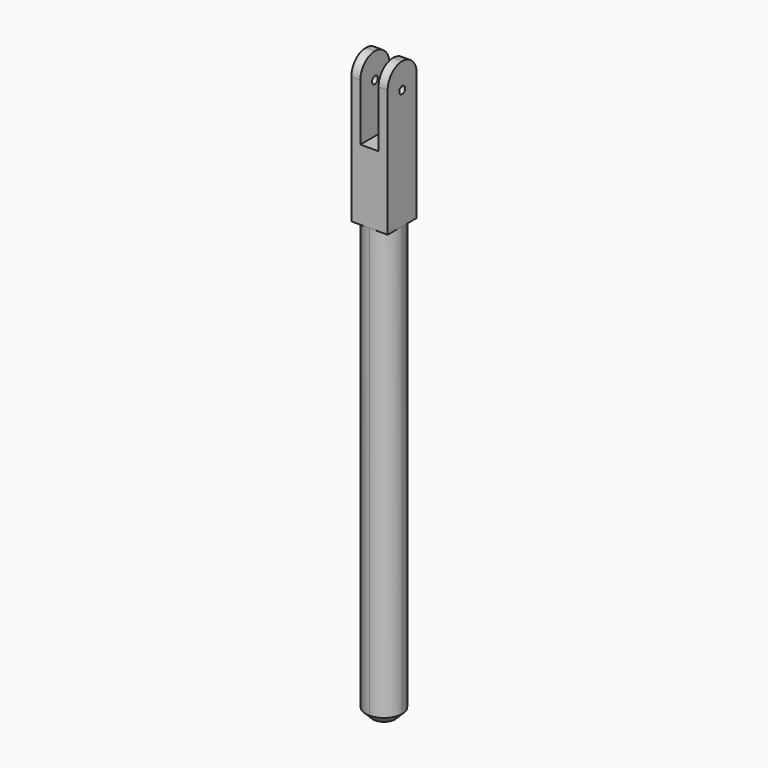
from build123d import *

# Parameters (mm, degrees)
F0_W     = 6.35
F0_H     = 76.2
F1_DEPTH = 3.175
F2_R     = 3.17499
F3_W     = 6.35
F3_H     = 25.4
F5_DEPTH = 3.175
F4_W     = 3.175
F4_H     = 13.0743015936
F6_DEPTH = 5.08
F7_R     = 0.635
F8_DEPTH = 3.81
F9_R     = 3.17499
F10_SIZE = 1.27


# Not quite as in the source:
# - a fillet or chamfer is up to 0.001 mm smaller than in the source, because OpenCascade refuses the exact size


with BuildPart() as f1:
    # F0 (on Front) → F1 (new body, symmetric)
    with BuildSketch(Plane.XZ):
        with Locations((-0.5868453211, -38.1)):
            Rectangle(F0_W, F0_H)
    extrude(amount=F1_DEPTH, both=True)

    # F2 (radius 3.175 in the source; OpenCascade refuses exactly that, so slightly less here)
    f2_edges = [f1.edges().sort_by_distance(p)[0] for p in [
        (2.588155, -3.175, -38.1),
        (2.588155, 3.175, -38.1),
        (-3.761845, -3.175, -38.1),
        (-3.761845, 3.175, -38.1),
    ]]
    fillet(f2_edges, radius=F2_R)

    # F3 (on Front) → F5 (join, symmetric)
    with BuildSketch(Plane.XZ):
        with Locations((-0.5868453211, 12.7)):
            Rectangle(F3_W, F3_H)
    extrude(amount=F5_DEPTH, both=True)

    # F4 (on Front) → F6 (cut, symmetric)
    with BuildSketch(Plane.XZ):
        with Locations((-0.5868453211, 18.8628492032)):
            Rectangle(F4_W, F4_H)
    extrude(amount=F6_DEPTH, both=True, mode=Mode.SUBTRACT)

    # F7 (on Right) → F8 (cut, symmetric)
    with BuildSketch(Plane.YZ):
        with Locations((0, 20.955)):
            Circle(F7_R)
    extrude(amount=F8_DEPTH, both=True, mode=Mode.SUBTRACT)

    # F9 (radius 3.175 in the source; OpenCascade refuses exactly that, so slightly less here)
    f9_edges = [f1.edges().sort_by_distance(p)[0] for p in [
        (-2.968095, -3.175, 25.4),
        (1.794405, -3.175, 25.4),
        (1.794405, 3.175, 25.4),
        (-2.968095, 3.175, 25.4),
    ]]
    fillet(f9_edges, radius=F9_R)

    # F10
    f10_edges = [f1.edges().sort_by_distance(p)[0] for p in [
        (-2.831912, 2.245067, -76.2),
    ]]
    chamfer(f10_edges, length=F10_SIZE)


solid = f1.part
